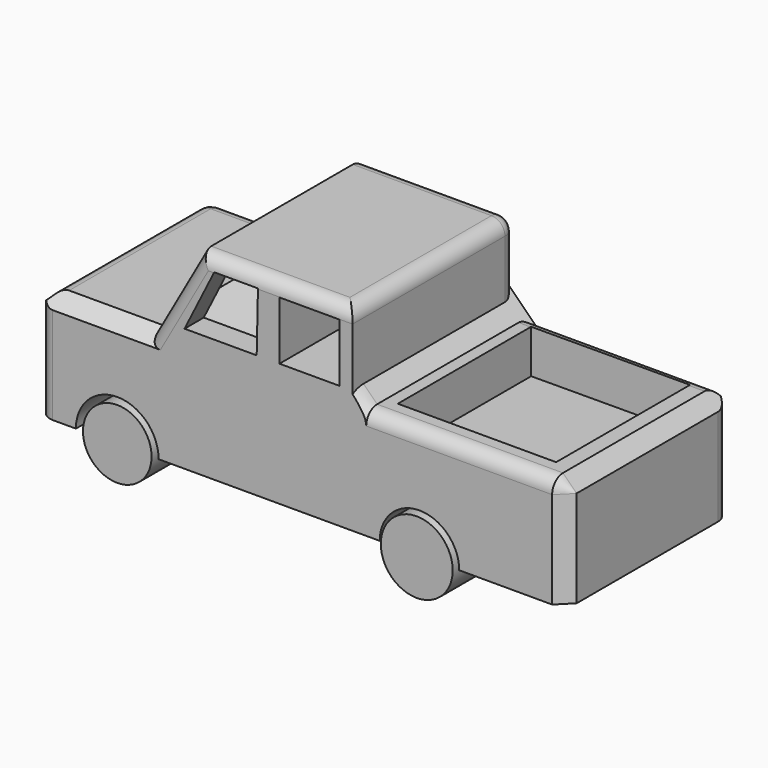
from build123d import *

# Parameters (mm, degrees)
F1_DEPTH      = 76.2
F2_T1_DEPTH   = 82.2454749882
F2_T3_DEPTH   = 101.6
F2_T8_DEPTH   = 61.9240448763
F3_SIZE       = 5.08
F4_R          = 5.08
F5_R          = 5.08
F6_T1_DEPTH   = 71.12
F6_T6_ANGLE   = 237.4057717794
F6_T8_DEPTH   = 49.1971181071
F6_T10_DEPTH  = 84.1841495789
F6_T13_ANGLE  = 90
F8_DEPTH      = 30.48
F10_DEPTH     = 25.4
F12_R         = 15.4477433976
F12_R_2       = 12.8167131571
F13_DEPTH     = 76.2
F14_R         = 14.8497475739
F15_DEPTH     = 76.2
F16_DEPTH     = 76.2
F17_DEPTH     = 77.47
F18_T1_DEPTH  = 64.4654749882
F18_T6_DEPTH  = 61.9240448763
F18_T11_DEPTH = 67.7498786986
F18_T14_ANGLE = 90.0000000017
F18_T18_DEPTH = 34.3734642797
F18_T24_DEPTH = 67.7498786986
F18_T28_DEPTH = 61.9240448763
F19_SIZE      = 5.07999
F20_T4_DEPTH  = 94.8236597681
F21_R         = 5.08
F22_R         = 5.08
F23_R         = 6.4459683432
F24_DEPTH     = 12.7
F25_R         = 5.5186924219
F26_DEPTH     = 12.7


# Not quite as in the source:
# - a fillet or chamfer that OpenCascade refuses, or shapes differently, is made with other operations: its cross-section is extruded or revolved along the edge and cut away or added
# - a fillet or chamfer is up to 0.001 mm smaller than in the source, because OpenCascade refuses the exact size
# - a feature names something its author has since deleted; it is built from what else it names
# - the program builds the solid bodies; features that only make, move or delete a surface that nothing else refers to are left out


with BuildPart() as f1:
    # F0 (on Front) → F1 (new body)
    with BuildSketch(Plane.XZ):
        with BuildLine():
            Line((-66.651314497, -14.2113678157), (-75.1781389117, -14.2113678157))
            Line((-75.1781389117, -14.2113678157), (-75.1781389117, -55.424336344))
            Line((-75.1781389117, -55.424336344), (-58.9820734658, -55.424336344))
            ThreePointArc((-58.9820734658, -55.424336344), (-45.9602549672, -42.4025178455), (-32.9384364687, -55.424336344))
            Line((-32.9384364687, -55.424336344), (53.461017087, -55.424336344))
            ThreePointArc((53.461017087, -55.424336344), (66.8888092041, -41.9965442269), (80.3166013212, -55.424336344))
            Line((80.3166013212, -55.424336344), (121.5071976185, -55.424336344))
            Line((121.5071976185, -55.424336344), (121.5071976185, -37.5180095434))
            Line((121.5071976185, -37.5180095434), (121.5071976185, -14.2113678157))
            Line((121.5071976185, -14.2113678157), (41.9235378504, -14.2113678157))
            Line((41.9235378504, -14.2113678157), (-32.8282602131, -14.2113678157))
            Line((-32.8282602131, -14.2113678157), (-66.651314497, -14.2113678157))
        make_face()
        Polygon((-14.9219371378, 17.622096464), (-32.8282602131, -14.2113678157), (41.9235378504, -14.2113678157), (41.9235378504, 17.622096464), align=None)
        Polygon((-20.8475716081, -9.3802222982), (-9.7422166161, 12.7864088863), (6.5759164281, 12.7864088863), (6.1049396172, -9.3802222982), align=None, mode=Mode.SUBTRACT)
        Polygon((14.6131906658, -9.3496078625), (14.6131906658, 12.4364411458), (37.0022393763, 12.4364411458), (37.1173098683, -9.3496078625), align=None, mode=Mode.SUBTRACT)
        with BuildLine():
            ThreePointArc((-32.9384364687, -55.424336344), (-45.9602549672, -42.4025178455), (-58.9820734658, -55.424336344))
            Line((-58.9820734658, -55.424336344), (-32.9384364687, -55.424336344))
        make_face()
        with BuildLine():
            Line((-32.9384364687, -55.424336344), (-58.9820734658, -55.424336344))
            ThreePointArc((-58.9820734658, -55.424336344), (-45.9602549672, -68.4461548426), (-32.9384364687, -55.424336344))
        make_face()
        with BuildLine():
            ThreePointArc((80.3166013212, -55.424336344), (66.8888092041, -41.9965442269), (53.461017087, -55.424336344))
            Line((53.461017087, -55.424336344), (80.3166013212, -55.424336344))
        make_face()
        with BuildLine():
            Line((80.3166013212, -55.424336344), (53.461017087, -55.424336344))
            ThreePointArc((53.461017087, -55.424336344), (66.8888092041, -68.8521284611), (80.3166013212, -55.424336344))
        make_face()
    extrude(amount=F1_DEPTH)

    # F2: fillet of radius 5.08 on 3 edges, made by hand

    # F2_s2 → F2_t1 (cut)
    with BuildSketch(Plane.YZ.offset(-27.6219371378)):
        with BuildLine():
            ThreePointArc((-71.12, 17.622096464), (-74.7121024484, 16.1341989125), (-76.2, 12.542096464))
            Line((-76.2, 12.542096464), (-76.2, 17.622096464))
            Line((-76.2, 17.622096464), (-71.12, 17.622096464))
        make_face()
    extrude(amount=F2_T1_DEPTH, mode=Mode.SUBTRACT)

    # F2_s4 → F2_t3 (cut)
    with BuildSketch(Plane.XZ.offset(-12.7)):
        with BuildLine():
            ThreePointArc((41.9235378504, 12.542096464), (40.4356402988, 16.1341989125), (36.8435378504, 17.622096464))
            Line((36.8435378504, 17.622096464), (41.9235378504, 17.622096464))
            Line((41.9235378504, 17.622096464), (41.9235378504, 12.542096464))
        make_face()
    extrude(amount=F2_T3_DEPTH, mode=Mode.SUBTRACT)


with BuildPart() as f2_tool6:
    # F2_s7 → F2_t8 (new body)
    with BuildSketch(Plane(origin=(10.1696558671, 0, 18.0793887958), x_dir=(0, 1, 0), z_dir=(-0.4902612275, 0, -0.8715755439))):
        with BuildLine():
            ThreePointArc((-71.12, -21.6450261215), (-74.7121024484, -20.1571285699), (-76.2, -16.5650261215))
            Line((-76.2, -16.5650261215), (-76.2, -21.6450261215))
            Line((-76.2, -21.6450261215), (-71.12, -21.6450261215))
        make_face()
    extrude(amount=F2_T8_DEPTH)

    split(bisect_by=Plane.XY.offset(-14.2113678157), keep=Keep.TOP)


with BuildPart() as f1_1:
    add(f1.part)

    # F2_t5: cut F2_tool6
    add(f2_tool6.part, mode=Mode.SUBTRACT)

    # F3
    f3_edges = [f1_1.edges().sort_by_distance(p)[0] for p in [
        (-51.088937, -76.2, -14.211368),
    ]]
    chamfer(f3_edges, length=F3_SIZE)

    # F4
    f4_edges = [f1_1.edges().sort_by_distance(p)[0] for p in [
        (-75.178139, -76.2, -37.357852),
    ]]
    fillet(f4_edges, radius=F4_R)

    # F5
    f5_edges = [f1_1.edges().sort_by_distance(p)[0] for p in [
        (81.715368, -76.2, -14.211368),
    ]]
    fillet(f5_edges, radius=F5_R)

    # F6: chamfer of 5.08 on 4 edges, made by hand

    # F6_s2 → F6_t1 (join)
    with BuildSketch(Plane.XZ):
        Polygon((41.9235378504, -9.1313678157), (47.0035378504, -14.2113678157), (41.9235378504, -14.2113678157), align=None)
    extrude(amount=F6_T1_DEPTH)


with BuildPart() as f6_tool4:
    # F6_s5 → F6_t6 (revolve)
    with BuildSketch(Plane(origin=(0, -29.3930998832, -45.970911519), x_dir=(1, 0, 0), z_dir=(0, 0.5386859165, 0.8425066666))):
        Polygon((47.0035378504, -44.447085979), (41.9235378504, -39.367085979), (41.9235378504, -44.447085979), align=None)
    revolve(axis=Axis((41.9235378504, -71.12, -19.2913678157), (-1, 0, 0)), revolution_arc=F6_T6_ANGLE)

    split(bisect_by=Plane.XZ.offset(76.2), keep=Keep.BOTTOM)


with BuildPart() as f1_2:
    add(f1_1.part)

    # F6_t3: union F6_tool4
    add(f6_tool4.part)

    # F6_s9 → F6_t8 (cut)
    with BuildSketch(Plane.XY.offset(-68.4884859229)):
        Polygon((116.4271976185, -76.2), (121.5071976185, -71.12), (121.5071976185, -76.2), align=None)
    extrude(amount=F6_T8_DEPTH, mode=Mode.SUBTRACT)

    # F6_s11 → F6_t10 (cut)
    with BuildSketch(Plane.XZ.offset(-13.0641495789)):
        Polygon((116.4271976185, -14.2113678157), (121.5071976185, -19.2913678157), (121.5071976185, -14.2113678157), align=None)
    extrude(amount=F6_T10_DEPTH, mode=Mode.SUBTRACT)

    # F6_s12 → F6_t13 (revolve, cut)
    with BuildSketch(Plane.XY.offset(-19.2913678157)):
        Polygon((116.4271976185, -76.2), (121.5071976185, -71.12), (121.5071976185, -76.2), align=None)
    revolve(axis=Axis((121.5071976185, -71.12, -19.2913678157), (-1, 0, 0)), revolution_arc=F6_T13_ANGLE, mode=Mode.SUBTRACT)

    # F7 (on Top) → F8 (cut)
    with BuildSketch(Plane.XY):
        Polygon((110.6219664216, -4.5476378873), (51.502674818, -4.8318649642), (51.502674818, -67.0776590705), (110.6219664216, -67.0776590705), align=None)
    extrude(amount=-F8_DEPTH, mode=Mode.SUBTRACT)

    # F9 (on face) → F10 (cut)
    with BuildSketch(Plane(origin=(-18.8652754153, 0, 10.6117170762), x_dir=(0, -1, 0), z_dir=(-0.8715755439, 0, 0.4902612275))):
        Polygon((4.4055245817, 3.4778357949), (4.6897507273, 0), (4.6897507273, -24.8935203999), (67.2197714448, -24.8935203999), (67.2197714448, 3.4778357949), align=None)
    extrude(amount=-F10_DEPTH, mode=Mode.SUBTRACT)

    # F12 (on face) → F13 (cut)
    with BuildSketch(Plane.XZ.offset(76.2)):
        with Locations((-45.9602549672, -55.424336344)):
            Circle(F12_R)
        with Locations((-45.9602549672, -55.424336344)):
            Circle(F12_R_2, mode=Mode.SUBTRACT)
    extrude(amount=-F13_DEPTH, mode=Mode.SUBTRACT)

    # F14 (on face) → F15 (cut)
    with BuildSketch(Plane.XZ.offset(76.2)):
        with Locations((66.8888092041, -55.424336344)):
            Circle(F14_R)
    extrude(amount=-F15_DEPTH, mode=Mode.SUBTRACT)

    # F14 (on face) → F16 (cut)
    with BuildSketch(Plane.XZ.offset(76.2)):
        with Locations((66.8888092041, -55.424336344)):
            Circle(F14_R)
    extrude(amount=-F16_DEPTH, mode=Mode.SUBTRACT)

    # F18: fillet of radius 5.08 on 3 edges, made by hand

    # F18_s2 → F18_t1 (cut)
    with BuildSketch(Plane.YZ.offset(-27.6219371378)):
        with BuildLine():
            ThreePointArc((0, 12.542096464), (-1.4878975516, 16.1341989125), (-5.08, 17.622096464))
            Line((-5.08, 17.622096464), (0, 17.622096464))
            Line((0, 17.622096464), (0, 12.542096464))
        make_face()
    extrude(amount=F18_T1_DEPTH, mode=Mode.SUBTRACT)


with BuildPart() as f17:
    # F0 (on Front) → F17 (new body)
    with BuildSketch(Plane.XZ):
        with BuildLine():
            Line((80.3166013212, -55.424336344), (53.461017087, -55.424336344))
            ThreePointArc((53.461017087, -55.424336344), (66.8888092041, -68.8521284611), (80.3166013212, -55.424336344))
        make_face()
        with BuildLine():
            ThreePointArc((80.3166013212, -55.424336344), (66.8888092041, -41.9965442269), (53.461017087, -55.424336344))
            Line((53.461017087, -55.424336344), (80.3166013212, -55.424336344))
        make_face()
    extrude(amount=F17_DEPTH)


with BuildPart() as f18_tool4:
    # F18_s5 → F18_t6 (new body)
    with BuildSketch(Plane(origin=(10.1696558671, 0, 18.0793887958), x_dir=(0, 1, 0), z_dir=(-0.4902612275, 0, -0.8715755439))):
        with BuildLine():
            ThreePointArc((0, -16.5650261215), (-1.4878975516, -20.1571285699), (-5.08, -21.6450261215))
            Line((-5.08, -21.6450261215), (0, -21.6450261215))
            Line((0, -21.6450261215), (0, -16.5650261215))
        make_face()
    extrude(amount=F18_T6_DEPTH)

    split(bisect_by=Plane.XY.offset(-14.2113678157), keep=Keep.TOP)


with BuildPart() as f1_3:
    add(f1_2.part)

    # F18_t3: cut F18_tool4
    add(f18_tool4.part, mode=Mode.SUBTRACT)


with BuildPart() as f18_tool9:
    # F18_s10 → F18_t11 (new body)
    with BuildSketch(Plane.YZ.offset(-20.1282602131)):
        with BuildLine():
            ThreePointArc((0, -19.2913678157), (-1.4878975516, -15.6992653673), (-5.08, -14.2113678157))
            Line((-5.08, -14.2113678157), (0, -14.2113678157))
            Line((0, -14.2113678157), (0, -19.2913678157))
        make_face()
    extrude(amount=-F18_T11_DEPTH)

    split(bisect_by=Plane(origin=(-18.8652754153, 0, 10.6117170762), x_dir=(0, 1, 0), z_dir=(-0.8715755439, 0, 0.4902612275)), keep=Keep.TOP)


with BuildPart() as f1_4:
    add(f1_3.part)

    # F18_t8: cut F18_tool9
    add(f18_tool9.part, mode=Mode.SUBTRACT)

    # F18_s13 → F18_t14 (revolve, cut)
    with BuildSketch(Plane.YZ.offset(36.8435378505)):
        with BuildLine():
            ThreePointArc((0, 12.542096464), (-1.4878975516, 16.1341989124), (-5.08, 17.622096464))
            Line((-5.08, 17.622096464), (0, 17.622096464))
            Line((0, 17.622096464), (0, 12.542096464))
        make_face()
    revolve(axis=Axis((36.8435378505, 0, 12.5420964641), (0, 1, 0)), revolution_arc=F18_T14_ANGLE, mode=Mode.SUBTRACT)


with BuildPart() as f18_tool16:
    # F18_s17 → F18_t18 (new body)
    with BuildSketch(Plane.XY.offset(-21.8313678157)):
        with BuildLine():
            ThreePointArc((41.9235378504, -5.08), (40.4356402988, -1.4878975516), (36.8435378504, 0))
            Line((36.8435378504, 0), (41.9235378504, 0))
            Line((41.9235378504, 0), (41.9235378504, -5.08))
        make_face()
    extrude(amount=F18_T18_DEPTH)

    split(bisect_by=Plane(origin=(16.3960850174, 0, 16.3960850174), x_dir=(0, 1, 0), z_dir=(0.7071067812, 0, 0.7071067812)), keep=Keep.TOP)


with BuildPart() as f1_5:
    add(f1_4.part)

    # F18_t15: cut F18_tool16
    add(f18_tool16.part, mode=Mode.SUBTRACT)


with BuildPart() as f18_tool22:
    # F18_s23 → F18_t24 (new body)
    with BuildSketch(Plane.YZ.offset(-20.1282602131)):
        with BuildLine():
            ThreePointArc((0, -19.2913678157), (-1.4878975516, -15.6992653673), (-5.08, -14.2113678157))
            Line((-5.08, -14.2113678157), (0, -14.2113678157))
            Line((0, -14.2113678157), (0, -19.2913678157))
        make_face()
    extrude(amount=-F18_T24_DEPTH)

    split(bisect_by=Plane(origin=(-18.8652754153, 0, 10.6117170762), x_dir=(0, 1, 0), z_dir=(0.8715755439, 0, -0.4902612275)), keep=Keep.TOP)


with BuildPart() as f18_tool26:
    # F18_s27 → F18_t28 (new body)
    with BuildSketch(Plane(origin=(10.1696558671, 0, 18.0793887958), x_dir=(0, 1, 0), z_dir=(-0.4902612275, 0, -0.8715755439))):
        with BuildLine():
            ThreePointArc((0, -16.5650261215), (-1.4878975516, -20.1571285699), (-5.08, -21.6450261215))
            Line((-5.08, -21.6450261215), (0, -21.6450261215))
            Line((0, -21.6450261215), (0, -16.5650261215))
        make_face()
    extrude(amount=F18_T28_DEPTH)

    split(bisect_by=Plane.XY.offset(-14.2113678157), keep=Keep.BOTTOM)


with BuildPart() as f18_tool22_1:
    add(f18_tool22.part)

    # F18_t30: intersect F18_tool26
    add(f18_tool26.part, mode=Mode.INTERSECT)


with BuildPart() as f1_6:
    add(f1_5.part)

    # F18_t20: cut F18_tool22
    add(f18_tool22_1.part, mode=Mode.SUBTRACT)

    # F19 (size 5.08 in the source; OpenCascade refuses exactly that, so slightly less here)
    f19_edges = [f1_6.edges().sort_by_distance(p)[0] for p in [
        (-75.178139, 0, -37.357852),
    ]]
    chamfer(f19_edges, length=F19_SIZE)

    # F20: fillet of radius 5.08 on 2 edges, made by hand


with BuildPart() as f20_tool2:
    # F20_s3 → F20_t4 (new body)
    with BuildSketch(Plane.YZ.offset(129.1271976185)):
        with BuildLine():
            ThreePointArc((0, -19.2913678157), (-1.4878975516, -15.6992653673), (-5.08, -14.2113678157))
            Line((-5.08, -14.2113678157), (0, -14.2113678157))
            Line((0, -14.2113678157), (0, -19.2913678157))
        make_face()
    extrude(amount=-F20_T4_DEPTH)

    split(bisect_by=Plane(origin=(16.3960850173, 0, 16.3960850173), x_dir=(0, 1, 0), z_dir=(0.7071067812, 0, 0.7071067812)), keep=Keep.TOP)


with BuildPart() as f1_7:
    add(f1_6.part)

    # F20_t1: cut F20_tool2
    add(f20_tool2.part, mode=Mode.SUBTRACT)

    # F21
    f21_edges = [f1_7.edges().sort_by_distance(p)[0] for p in [
        (121.507198, 0, -37.357852),
    ]]
    fillet(f21_edges, radius=F21_R)

    # F22
    f22_edges = [f1_7.edges().sort_by_distance(p)[0] for p in [
        (-70.098149, 0, -37.357852),
        (-70.098149, -1.487898, -15.699265),
        (-70.098149, -38.1, -14.211368),
    ]]
    fillet(f22_edges, radius=F22_R)

    # F23 (on face) → F24 (cut)
    with BuildSketch(Plane(origin=(-75.1781389117, 0, 0), x_dir=(0, -1, 0), z_dir=(-1, 0, 0))):
        with Locations((18.1149821728, -37.3578520799)):
            Circle(F23_R)
    extrude(amount=-F24_DEPTH, mode=Mode.SUBTRACT)

    # F25 (on face) → F26 (cut)
    with BuildSketch(Plane(origin=(-75.1781389117, 0, 0), x_dir=(0, -1, 0), z_dir=(-1, 0, 0))):
        with Locations((59.896402061, -37.5180095434)):
            Circle(F25_R)
    extrude(amount=-F26_DEPTH, mode=Mode.SUBTRACT)


solid = Compound([f17.part, f1_7.part])
